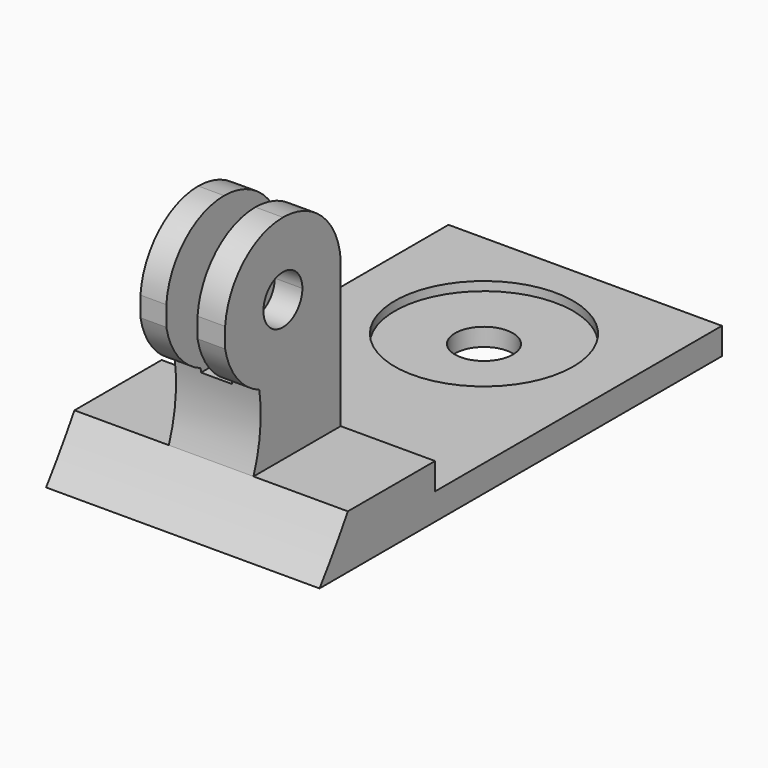
from build123d import *

# Parameters (mm, degrees)
F0_W      = 30.6736361235
F0_H      = 84.459155798
F0_R      = 3.25
F1_DEPTH  = 3
F2_W      = 30.6736361235
F2_H      = 16.2
F3_DEPTH  = 3
F4_W      = 9.5
F4_H      = 16.2
F5_DEPTH  = 24
F6_W      = 3.5
F6_H      = 16.2452395454
F7_DEPTH  = 18
F9_DEPTH  = 10
F10_R     = 10
F10_R_2   = 3.25
F11_DEPTH = 1
F12_W     = 30.6736361235
F12_H     = 28.0341655016
F13_DEPTH = 5
F15_DEPTH = 30.6746361235


# Not quite as in the source:
# - a feature names something its author has since deleted; it is built from what else it names


with BuildPart() as f1:
    # F0 (on Top) → F1 (new body)
    with BuildSketch(Plane.XY):
        Rectangle(F0_W, F0_H)
        Circle(F0_R, mode=Mode.SUBTRACT)
    extrude(amount=F1_DEPTH)

    # F2 (on face) → F3 (join)
    with BuildSketch(Plane.XY.offset(3)):
        with Locations((0, -34.129577899)):
            Rectangle(F2_W, F2_H)
    extrude(amount=F3_DEPTH)

    # F4 (on face) → F5 (join)
    with BuildSketch(Plane.XY.offset(6)):
        with Locations((0, -34.129577899)):
            Rectangle(F4_W, F4_H)
    extrude(amount=F5_DEPTH)

    # F6 (on face) → F7 (cut)
    with BuildSketch(Plane(origin=(0, -26.029577899, 0), x_dir=(-1, 0, 0), z_dir=(0, 1, 0))):
        with Locations((0.0963514363, 21.8773802273)):
            Rectangle(F6_W, F6_H)
    extrude(amount=-F7_DEPTH, mode=Mode.SUBTRACT)

    # F8 (on face) → F9 (cut)
    with BuildSketch(Plane.YZ.offset(4.75)):
        with BuildLine():
            Line((-26.029577899, 30), (-34.129577899, 30))
            Line((-34.129577899, 30), (-34.129577899, 29.9113391646))
            ThreePointArc((-34.129577899, 29.9113391646), (-28.6200020152, 27.7584969737), (-26.029577899, 22.440615928))
            Line((-26.029577899, 22.440615928), (-26.029577899, 30))
        make_face()
        with BuildLine():
            Line((-34.129577899, 29.9113391646), (-34.129577899, 30))
            Line((-34.129577899, 30), (-42.229577899, 30))
            Line((-42.229577899, 30), (-42.229577899, 22.440615928))
            ThreePointArc((-42.229577899, 22.440615928), (-39.6391537828, 27.7584969737), (-34.129577899, 29.9113391646))
        make_face()
        with BuildLine():
            ThreePointArc((-31.4004653301, 21.7848364264), (-32.1998038949, 23.7146104305), (-34.129577899, 24.5139489953))
            ThreePointArc((-34.129577899, 24.5139489953), (-36.0593519031, 19.8550624223), (-31.4004653301, 21.7848364264))
        make_face()
    extrude(amount=-F9_DEPTH, mode=Mode.SUBTRACT)

    # F10 (on face) → F11 (cut)
    with BuildSketch(Plane.XY.offset(3)):
        Circle(F10_R)
        Circle(F10_R_2, mode=Mode.SUBTRACT)
    extrude(amount=-F11_DEPTH, mode=Mode.SUBTRACT)

    # F12 (on face) → F13 (cut)
    with BuildSketch(Plane.XY.offset(3)):
        with Locations((0, 28.2124951482)):
            Rectangle(F12_W, F12_H)
    extrude(amount=-F13_DEPTH, mode=Mode.SUBTRACT)

    # F14 (on face) → F15 (cut, through all)
    with BuildSketch(Plane(origin=(-15.3368180618, 0, 0), x_dir=(0, -1, 0), z_dir=(-1, 0, 0))):
        with BuildLine():
            Line((38.2532812655, 6), (42.229577899, 6))
            Line((42.229577899, 6), (42.229577899, 20.2058496963))
            ThreePointArc((42.229577899, 20.2058496963), (40.5668907772, 16.6210972771), (37.4282303868, 14.220307964))
            ThreePointArc((37.4282303868, 14.220307964), (37.3242335364, 10.0583119864), (38.2532812655, 6))
        make_face()
        with BuildLine():
            Line((42.229577899, 0), (42.229577899, 6))
            Line((42.229577899, 6), (38.2532812655, 6))
            ThreePointArc((38.2532812655, 6), (40.1731353083, 2.9547402847), (42.229577899, 0))
        make_face()
    extrude(amount=-F15_DEPTH, mode=Mode.SUBTRACT)


solid = f1.part
